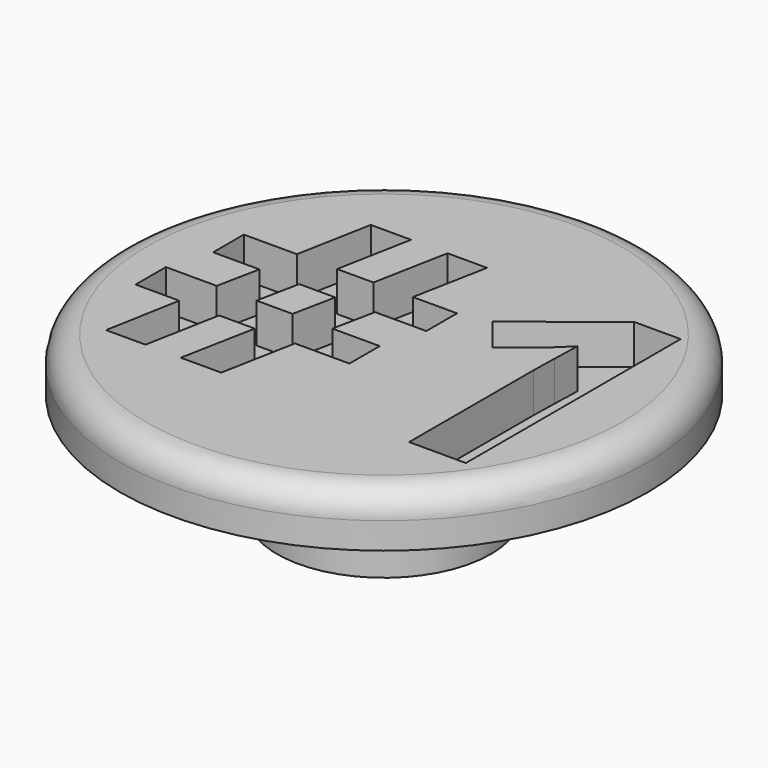
from build123d import *

# Parameters (mm, degrees)
F0_R         = 4.05
F1_DEPTH     = 6
F0_R_2       = 5
F2_DEPTH     = 2.5
F0_R_3       = 10
F3_DEPTH     = 2
F4_R         = 1
F5_TEXT_SIZE = 14.2360628389
F6_DEPTH     = 1.5


# Not quite as in the source:
# - Text() gives the source's letters only with a copy of the font that has no kerning and outlines rounded to 1/6400 em; it was checked with that copy


with BuildPart() as f1:
    # F0 (on Top) → F1 (new body)
    with BuildSketch(Plane.XY):
        Circle(F0_R)
    extrude(amount=-F1_DEPTH)

    # F0 (on Top) → F2 (join)
    with BuildSketch(Plane.XY):
        Circle(F0_R_2)
        Circle(F0_R, mode=Mode.SUBTRACT)
    extrude(amount=-F2_DEPTH)

    # F0 (on Top) → F3 (join)
    with BuildSketch(Plane.XY):
        Circle(F0_R_3)
        Circle(F0_R_2, mode=Mode.SUBTRACT)
    extrude(amount=-F3_DEPTH)

    # F4
    f4_edges = [f1.edges().sort_by_distance(p)[0] for p in [
        (-10, 0, 0),
    ]]
    fillet(f4_edges, radius=F4_R)

    # F5 (on Top) → F6 (cut)
    with BuildSketch(Plane.XY):
        with Locations((-8.0489774161, -4.9095719435)):
            Text('#1', F5_TEXT_SIZE, font='Open Sans', font_style=FontStyle.BOLD, text_align=(TextAlign.LEFT, TextAlign.BOTTOM))
    extrude(amount=-F6_DEPTH, mode=Mode.SUBTRACT)


solid = f1.part
